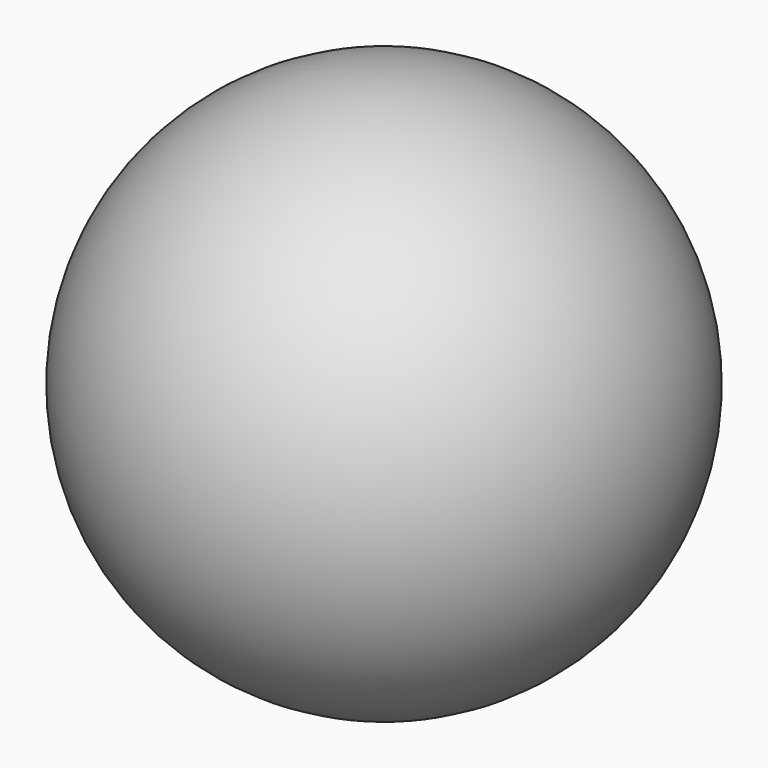
from build123d import *

# Parameters (mm, degrees)
F4_R         = 3.175
F5_DEPTH     = 38.1
F6_TEXT_SIZE = 3.6323591808
F7_DEPTH     = 31.75
F9_ANGLE     = -104.45


# Not quite as in the source:
# - Text() gives the source's letters only with a copy of the font that has no kerning and outlines rounded to 1/6400 em; it was checked with that copy


with BuildPart() as f2:
    # F1 (on Front) → F2 (revolve)
    with BuildSketch(Plane.XZ):
        with BuildLine():
            Line((0, -15.875), (0, 15.875))
            ThreePointArc((0, 15.875), (-15.875, 0), (0, -15.875))
        make_face()
    revolve(axis=Axis((0, 0, 0), (0, 0, 1)))

    # F6 (on face) → F7 (cut)
    with BuildSketch(Plane(origin=(0, 44.45, 0), x_dir=(-1, 0, 0), z_dir=(0, 1, 0))):
        with Locations((-4.653544187, 4.386571236)):
            Text('104.45', F6_TEXT_SIZE, font='Open Sans', text_align=(TextAlign.LEFT, TextAlign.BOTTOM))
    extrude(amount=-F7_DEPTH, mode=Mode.SUBTRACT)


with BuildPart() as f5:
    # F4 (on offset) → F5 (new body)
    with BuildSketch(Plane.XZ.offset(-6.35)):
        with Locations((-1.5955890995, 0)):
            Circle(F4_R)
    extrude(amount=-F5_DEPTH)


with BuildPart() as f9_1:
    # F9: copy of F5
    add(f5.part.rotate(Axis((19.8181457818, 0, 0), (1, 0, 0)), F9_ANGLE))


with BuildPart() as f2_1:
    add(f2.part)

    # F10: cut F9_1, F5
    add(f9_1.part, mode=Mode.SUBTRACT)
    add(f5.part, mode=Mode.SUBTRACT)


solid = f2_1.part
